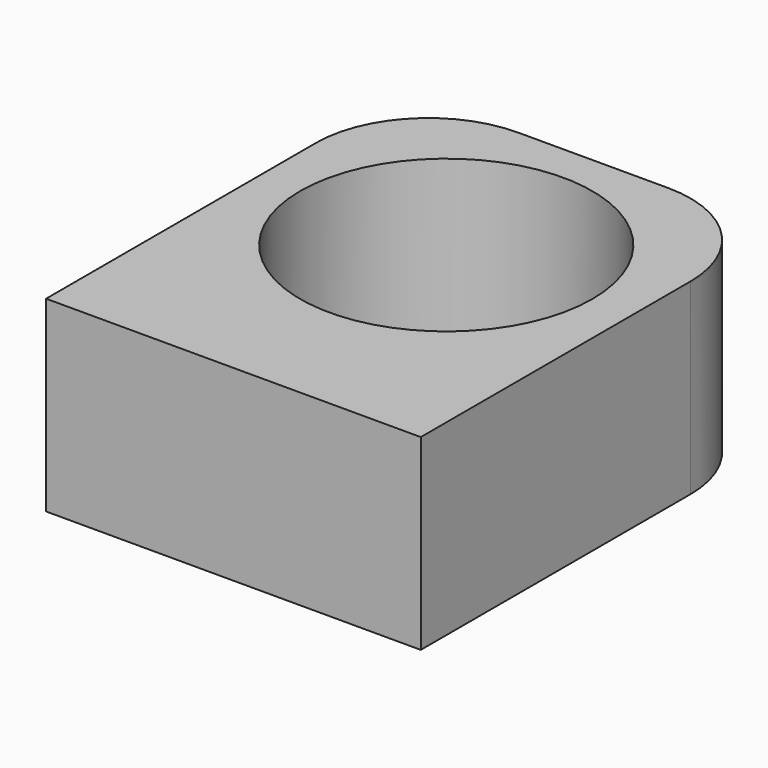
from build123d import *

# Parameters (mm, degrees)
F0_W     = 50
F0_H     = 60
F0_R     = 19.5
F1_DEPTH = 25
F2_R     = 15
F3_R     = 15


with BuildPart() as f1:
    # F0 (on Top) → F1 (new body)
    with BuildSketch(Plane.XY):
        Rectangle(F0_W, F0_H)
        with Locations((0, 5.5)):
            Circle(F0_R, mode=Mode.SUBTRACT)
    extrude(amount=F1_DEPTH)

    # F2
    f2_edges = [f1.edges().sort_by_distance(p)[0] for p in [
        (-25, 30, 12.5),
    ]]
    fillet(f2_edges, radius=F2_R)

    # F3
    f3_edges = [f1.edges().sort_by_distance(p)[0] for p in [
        (25, 30, 12.5),
    ]]
    fillet(f3_edges, radius=F3_R)


solid = f1.part
